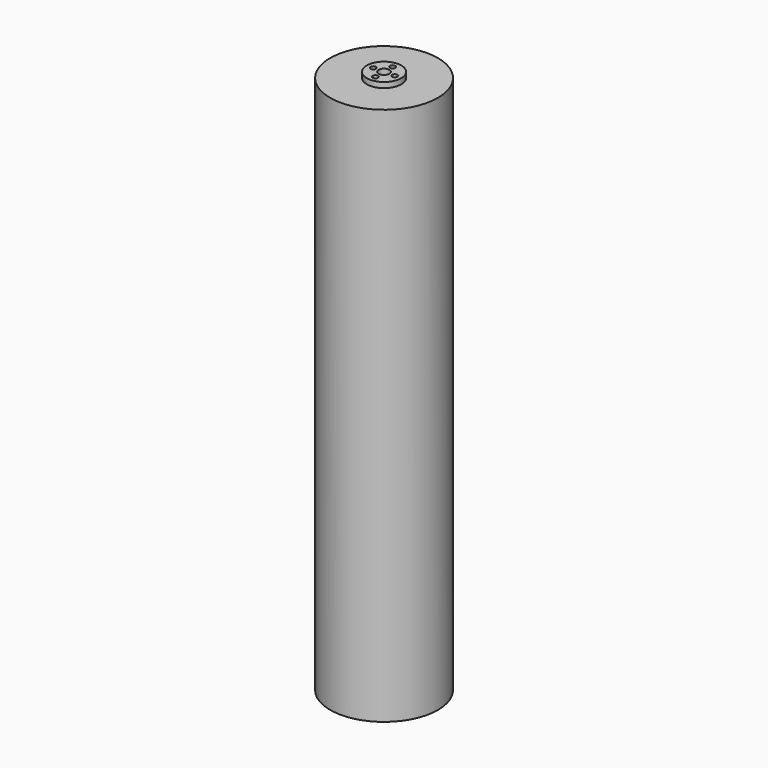
from build123d import *

# Parameters (mm, degrees)
F0_R      = 12
F0_R_2    = 10
F1_DEPTH  = 1000
F2_R      = 32
F2_R_2    = 12
F2_R_3    = 10
F3_DEPTH  = 10
F4_R      = 32
F4_R_2    = 12
F4_R_3    = 10
F5_DEPTH  = 10
F6_DEPTH  = 1000
F7_R      = 5
F8_DEPTH  = 5
F9_R      = 5
F10_DEPTH = 5
F11_R     = 100
F11_R_2   = 32
F12_DEPTH = 1000


with BuildPart() as f1:
    # F0 (on Top) → F1 (new body)
    with BuildSketch(Plane.XY):
        Circle(F0_R)
        Circle(F0_R_2, mode=Mode.SUBTRACT)
    extrude(amount=F1_DEPTH)


with BuildPart() as f3:
    # F2 (on face) → F3 (new body)
    with BuildSketch(Plane.XY.offset(1000)):
        Circle(F2_R)
        Circle(F2_R_2, mode=Mode.SUBTRACT)
        Circle(F2_R_2)
        Circle(F2_R_3, mode=Mode.SUBTRACT)
    extrude(amount=F3_DEPTH)


with BuildPart() as f5:
    # F4 (on face) → F5 (new body)
    with BuildSketch(Plane(origin=(0, 0, 0), x_dir=(1, 0, 0), z_dir=(0, 0, -1))):
        Circle(F4_R)
        Circle(F4_R_2, mode=Mode.SUBTRACT)
        Circle(F4_R_2)
        Circle(F4_R_3, mode=Mode.SUBTRACT)
    extrude(amount=F5_DEPTH)

    # F7 (on face) → F8 (cut)
    with BuildSketch(Plane(origin=(0, 0, -10), x_dir=(1, 0, 0), z_dir=(0, 0, -1))):
        with Locations((0, 20)):
            Circle(F7_R)
        with Locations((-20, 0)):
            Circle(F7_R)
        with Locations((0, -20)):
            Circle(F7_R)
        with Locations((20, 0)):
            Circle(F7_R)
    extrude(amount=-F8_DEPTH, mode=Mode.SUBTRACT)


with BuildPart() as f6:
    # F6 (new, through all): a face of the model
    f6_faces = [f3.part.faces().sort_by_distance(p)[0] for p in [
        (-31.0949033201, 0, 1000),
    ]]
    extrude(f6_faces, amount=F6_DEPTH)


with BuildPart() as f3_1:
    add(f3.part)

    # F9 (on face) → F10 (cut)
    with BuildSketch(Plane.XY.offset(1010)):
        with Locations((0, 20)):
            Circle(F9_R)
        with Locations((-20, 0)):
            Circle(F9_R)
        with Locations((0, -20)):
            Circle(F9_R)
        with Locations((20, 0)):
            Circle(F9_R)
    extrude(amount=-F10_DEPTH, mode=Mode.SUBTRACT)


with BuildPart() as f12:
    # F11 (on face) → F12 (new body, through all)
    with BuildSketch(Plane(origin=(0, 0, 1000), x_dir=(1, 0, 0), z_dir=(0, 0, -1))):
        Circle(F11_R)
        Circle(F11_R_2, mode=Mode.SUBTRACT)
    extrude(amount=F12_DEPTH)


solid = Compound([f1.part, f5.part, f6.part, f3_1.part, f12.part])
